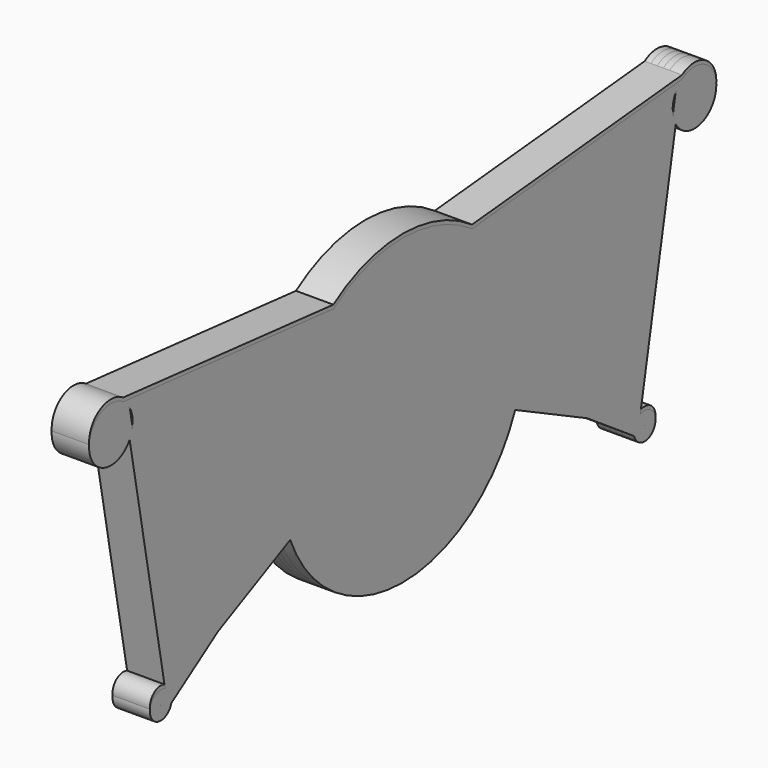
from build123d import *

# Parameters (mm, degrees)
F0_R     = 0.135
F0_R_2   = 0.27
F1_DEPTH = 25.4
F2_DEPTH = 6.35
F5_DEPTH = 12.7


# Not quite as in the source:
# - a feature of the source that left no trace in its solid (it failed there, or was rolled back) is left out


with BuildPart() as f1:
    # F0 (on Right) → F1 (new body)
    with BuildSketch(Plane.YZ):
        with BuildLine():
            ThreePointArc((148.1493894295, -44.1035673814), (152.9600066404, -22.2845823986), (154.5747917486, 0))
            ThreePointArc((154.5747917486, 0), (148.5279407682, 42.8114126754), (130.8604844604, 82.273324054))
            ThreePointArc((130.8604844604, 82.273324054), (111.8407913587, 106.700532484), (88.3348162489, 126.8476506775))
            ThreePointArc((88.3348162489, 126.8476506775), (0, 154.5747917486), (-88.3348162489, 126.8476506775))
            ThreePointArc((-88.3348162489, 126.8476506775), (-111.8407913587, 106.700532484), (-130.8604844604, 82.273324054))
            ThreePointArc((-130.8604844604, 82.273324054), (-153.1483173405, 20.9513517433), (-148.1493894296, -44.1035673814))
            ThreePointArc((-148.1493894296, -44.1035673814), (-145.885013799, -51.0972503466), (-143.2906938672, -57.9753680037))
            ThreePointArc((-143.2906938672, -57.9753680037), (0, -154.5747917486), (143.2906938672, -57.9753680037))
            ThreePointArc((143.2906938672, -57.9753680037), (145.885013799, -51.0972503466), (148.1493894295, -44.1035673814))
        make_face()
        with BuildLine():
            ThreePointArc((130.8604844604, 82.273324054), (148.5279407682, 42.8114126754), (154.5747917486, 0))
            ThreePointArc((154.5747917486, 0), (152.9600066404, -22.2845823986), (148.1493894295, -44.1035673814))
            Line((148.1493894296, -44.1035673814), (235.1719274058, -102.7744833812))
            Line((235.1719274058, -102.7744833812), (296.116428963, -132.4895802702))
            ThreePointArc((296.116428963, -132.4895802702), (296.5182456961, -131.8315982378), (296.9560527921, -131.1969944335))
            Line((296.9560527921, -131.1969944335), (344.4860615971, 123.2635601256))
            ThreePointArc((344.4860615971, 123.2635601256), (344.0765910751, 125.5101069455), (343.8526480641, 127.7826579901))
            Line((343.8526480641, 127.7826579901), (130.8604844604, 82.273324054))
        make_face()
        with BuildLine():
            ThreePointArc((88.3348162489, 126.8476506775), (111.8407913587, 106.700532484), (130.8604844604, 82.273324054))
            Line((130.8604844604, 82.273324054), (343.8526480641, 127.7826579901))
            ThreePointArc((343.8526480641, 127.7826579901), (344.791373956, 136.7102752623), (348.5227758692, 144.8748448298))
            ThreePointArc((348.5227758692, 144.8748448298), (351.8507398842, 148.9464286566), (355.885083858, 152.3194403742))
            Line((355.885083858, 152.3194403742), (88.3348162489, 126.8476506775))
        make_face()
        with BuildLine():
            Line((235.1719274058, -102.7744833812), (148.1493894296, -44.1035673814))
            ThreePointArc((148.1493894295, -44.1035673814), (145.885013799, -51.0972503466), (143.2906938672, -57.9753680037))
            Line((143.2906938672, -57.9753680037), (235.1719274058, -102.7744833812))
        make_face()
        with BuildLine():
            Line((296.116428963, -132.4895802702), (235.1719274058, -102.7744833812))
            Line((235.1719274058, -102.7744833812), (294.7499277685, -142.94219092))
            ThreePointArc((294.7499277685, -142.94219092), (294.3998362612, -137.5807936771), (296.116428963, -132.4895802702))
        make_face()
        with BuildLine():
            ThreePointArc((-130.8604844604, 82.273324054), (-111.8407913587, 106.700532484), (-88.3348162489, 126.8476506775))
            Line((-88.3348162489, 126.8476506775), (-355.885083858, 152.3194403742))
            ThreePointArc((-355.885083858, 152.3194403742), (-351.8507398842, 148.9464286566), (-348.5227758692, 144.8748448298))
            ThreePointArc((-348.5227758692, 144.8748448298), (-345.012126575, 137.4750271925), (-343.807133589, 129.3737957161))
            ThreePointArc((-343.807133589, 129.3737957161), (-343.8185145344, 128.5779014344), (-343.8526480641, 127.7826579901))
            Line((-343.8526480641, 127.7826579901), (-130.8604844604, 82.273324054))
        make_face()
        with BuildLine():
            ThreePointArc((399.477133589, 129.3737957161), (384.6072742696, 154.0049213934), (355.885083858, 152.3194403742))
            ThreePointArc((355.885083858, 152.3194403742), (351.8507398842, 148.9464286566), (348.5227758692, 144.8748448298))
            Line((348.5227758692, 144.8748448298), (344.4860615971, 123.2635601256))
            ThreePointArc((344.4860615971, 123.2635601256), (345.8076274671, 119.0120623456), (347.7901304496, 115.0256539813))
            ThreePointArc((347.7901304496, 115.0256539813), (379.0874917944, 102.5530226811), (399.477133589, 129.3737957161))
        make_face()
        with Locations((371.642133589, 129.3737957161)):
            Circle(F0_R, mode=Mode.SUBTRACT)
        with BuildLine():
            ThreePointArc((347.7901304496, 115.0256539813), (345.8076274671, 119.0120623456), (344.4860615971, 123.2635601256))
            Line((344.4860615971, 123.2635601256), (296.9560527921, -131.1969944335))
            ThreePointArc((296.9560527921, -131.1969944335), (299.4978488517, -128.5476375988), (302.6464556404, -126.6592271201))
            Line((302.6464556404, -126.6592271201), (347.7901304496, 115.0256539813))
        make_face()
        with BuildLine():
            Line((-235.1719274058, -102.7744833812), (-143.2906938672, -57.9753680037))
            ThreePointArc((-143.2906938672, -57.9753680037), (-145.885013799, -51.0972503466), (-148.1493894296, -44.1035673814))
            Line((-148.1493894295, -44.1035673814), (-235.1719274058, -102.7744833812))
        make_face()
        with BuildLine():
            ThreePointArc((296.9560527921, -131.1969944335), (296.5182456961, -131.8315982378), (296.116428963, -132.4895802702))
            ThreePointArc((296.116428963, -132.4895802702), (294.3998362612, -137.5807936771), (294.7499277685, -142.94219092))
            ThreePointArc((294.7499277685, -142.94219092), (309.9312086468, -153.1089342258), (321.9829761036, -139.3761683092))
            ThreePointArc((321.9829761036, -139.3761683092), (315.7433043352, -127.8044180436), (302.6464556404, -126.6592271201))
            ThreePointArc((302.6464556404, -126.6592271201), (299.4978488517, -128.5476375988), (296.9560527921, -131.1969944335))
        make_face()
        with Locations((308.1329761036, -139.3761683092)):
            Circle(F0_R_2, mode=Mode.SUBTRACT)
        with BuildLine():
            ThreePointArc((-148.1493894296, -44.1035673814), (-153.1483173405, 20.9513517433), (-130.8604844604, 82.273324054))
            Line((-130.8604844604, 82.273324054), (-343.8526480641, 127.7826579901))
            ThreePointArc((-343.8526480641, 127.7826579901), (-344.0765910751, 125.5101069455), (-344.4860615971, 123.2635601256))
            Line((-344.4860615971, 123.2635601256), (-296.9560527921, -131.1969944335))
            ThreePointArc((-296.9560527921, -131.1969944335), (-296.5182456961, -131.8315982378), (-296.116428963, -132.4895802702))
            Line((-296.116428963, -132.4895802702), (-235.1719274058, -102.7744833812))
            Line((-235.1719274058, -102.7744833812), (-148.1493894295, -44.1035673814))
        make_face()
        with BuildLine():
            ThreePointArc((-348.5227758692, 144.8748448298), (-351.8507398842, 148.9464286566), (-355.885083858, 152.3194403742))
            ThreePointArc((-355.885083858, 152.3194403742), (-398.8437124622, 123.4694471661), (-347.7901304496, 115.0256539813))
            ThreePointArc((-347.7901304496, 115.0256539813), (-345.8076274671, 119.0120623456), (-344.4860615971, 123.2635601256))
            Line((-344.4860615971, 123.2635601256), (-348.5227758692, 144.8748448298))
        make_face()
        with Locations((-371.642133589, 129.3737957161)):
            Circle(F0_R, mode=Mode.SUBTRACT)
        with BuildLine():
            Line((-294.7499277685, -142.94219092), (-235.1719274058, -102.7744833812))
            Line((-235.1719274058, -102.7744833812), (-296.116428963, -132.4895802702))
            ThreePointArc((-296.116428963, -132.4895802702), (-294.7491859473, -135.8129308695), (-294.2829761036, -139.3761683092))
            ThreePointArc((-294.2829761036, -139.3761683092), (-294.400210187, -141.1744008524), (-294.7499277685, -142.94219092))
        make_face()
        with BuildLine():
            ThreePointArc((-344.4860615971, 123.2635601256), (-345.8076274671, 119.0120623456), (-347.7901304496, 115.0256539813))
            Line((-347.7901304496, 115.0256539813), (-302.6464556404, -126.6592271201))
            ThreePointArc((-302.6464556404, -126.6592271201), (-299.4978488517, -128.5476375988), (-296.9560527921, -131.1969944335))
            Line((-296.9560527921, -131.1969944335), (-344.4860615971, 123.2635601256))
        make_face()
        with BuildLine():
            ThreePointArc((-302.6464556404, -126.6592271201), (-320.5948733984, -145.4196454386), (-294.7499277685, -142.94219092))
            ThreePointArc((-294.7499277685, -142.94219092), (-294.400210187, -141.1744008524), (-294.2829761036, -139.3761683092))
            ThreePointArc((-294.2829761036, -139.3761683092), (-294.7491859473, -135.8129308695), (-296.116428963, -132.4895802702))
            ThreePointArc((-296.116428963, -132.4895802702), (-296.5182456961, -131.8315982378), (-296.9560527921, -131.1969944335))
            ThreePointArc((-296.9560527921, -131.1969944335), (-299.4978488517, -128.5476375988), (-302.6464556404, -126.6592271201))
        make_face()
        with Locations((-308.1329761036, -139.3761683092)):
            Circle(F0_R_2, mode=Mode.SUBTRACT)
    extrude(amount=F1_DEPTH)

    # F0 (on Right) → F2 (join, symmetric)
    with BuildSketch(Plane.YZ):
        with BuildLine():
            ThreePointArc((148.1493894295, -44.1035673814), (152.9600066404, -22.2845823986), (154.5747917486, 0))
            ThreePointArc((154.5747917486, 0), (148.5279407682, 42.8114126754), (130.8604844604, 82.273324054))
            ThreePointArc((130.8604844604, 82.273324054), (111.8407913587, 106.700532484), (88.3348162489, 126.8476506775))
            ThreePointArc((88.3348162489, 126.8476506775), (0, 154.5747917486), (-88.3348162489, 126.8476506775))
            ThreePointArc((-88.3348162489, 126.8476506775), (-111.8407913587, 106.700532484), (-130.8604844604, 82.273324054))
            ThreePointArc((-130.8604844604, 82.273324054), (-153.1483173405, 20.9513517433), (-148.1493894296, -44.1035673814))
            ThreePointArc((-148.1493894296, -44.1035673814), (-145.885013799, -51.0972503466), (-143.2906938672, -57.9753680037))
            ThreePointArc((-143.2906938672, -57.9753680037), (0, -154.5747917486), (143.2906938672, -57.9753680037))
            ThreePointArc((143.2906938672, -57.9753680037), (145.885013799, -51.0972503466), (148.1493894295, -44.1035673814))
        make_face()
        with BuildLine():
            ThreePointArc((130.8604844604, 82.273324054), (148.5279407682, 42.8114126754), (154.5747917486, 0))
            ThreePointArc((154.5747917486, 0), (152.9600066404, -22.2845823986), (148.1493894295, -44.1035673814))
            Line((148.1493894296, -44.1035673814), (235.1719274058, -102.7744833812))
            Line((235.1719274058, -102.7744833812), (296.116428963, -132.4895802702))
            ThreePointArc((296.116428963, -132.4895802702), (296.5182456961, -131.8315982378), (296.9560527921, -131.1969944335))
            Line((296.9560527921, -131.1969944335), (344.4860615971, 123.2635601256))
            ThreePointArc((344.4860615971, 123.2635601256), (344.0765910751, 125.5101069455), (343.8526480641, 127.7826579901))
            Line((343.8526480641, 127.7826579901), (130.8604844604, 82.273324054))
        make_face()
        with BuildLine():
            ThreePointArc((88.3348162489, 126.8476506775), (111.8407913587, 106.700532484), (130.8604844604, 82.273324054))
            Line((130.8604844604, 82.273324054), (343.8526480641, 127.7826579901))
            ThreePointArc((343.8526480641, 127.7826579901), (344.791373956, 136.7102752623), (348.5227758692, 144.8748448298))
            ThreePointArc((348.5227758692, 144.8748448298), (351.8507398842, 148.9464286566), (355.885083858, 152.3194403742))
            Line((355.885083858, 152.3194403742), (88.3348162489, 126.8476506775))
        make_face()
        with BuildLine():
            Line((235.1719274058, -102.7744833812), (148.1493894296, -44.1035673814))
            ThreePointArc((148.1493894295, -44.1035673814), (145.885013799, -51.0972503466), (143.2906938672, -57.9753680037))
            Line((143.2906938672, -57.9753680037), (235.1719274058, -102.7744833812))
        make_face()
        with BuildLine():
            Line((296.116428963, -132.4895802702), (235.1719274058, -102.7744833812))
            Line((235.1719274058, -102.7744833812), (294.7499277685, -142.94219092))
            ThreePointArc((294.7499277685, -142.94219092), (294.3998362612, -137.5807936771), (296.116428963, -132.4895802702))
        make_face()
        with BuildLine():
            ThreePointArc((-130.8604844604, 82.273324054), (-111.8407913587, 106.700532484), (-88.3348162489, 126.8476506775))
            Line((-88.3348162489, 126.8476506775), (-355.885083858, 152.3194403742))
            ThreePointArc((-355.885083858, 152.3194403742), (-351.8507398842, 148.9464286566), (-348.5227758692, 144.8748448298))
            ThreePointArc((-348.5227758692, 144.8748448298), (-345.012126575, 137.4750271925), (-343.807133589, 129.3737957161))
            ThreePointArc((-343.807133589, 129.3737957161), (-343.8185145344, 128.5779014344), (-343.8526480641, 127.7826579901))
            Line((-343.8526480641, 127.7826579901), (-130.8604844604, 82.273324054))
        make_face()
        with BuildLine():
            ThreePointArc((399.477133589, 129.3737957161), (384.6072742696, 154.0049213934), (355.885083858, 152.3194403742))
            ThreePointArc((355.885083858, 152.3194403742), (351.8507398842, 148.9464286566), (348.5227758692, 144.8748448298))
            Line((348.5227758692, 144.8748448298), (344.4860615971, 123.2635601256))
            ThreePointArc((344.4860615971, 123.2635601256), (345.8076274671, 119.0120623456), (347.7901304496, 115.0256539813))
            ThreePointArc((347.7901304496, 115.0256539813), (379.0874917944, 102.5530226811), (399.477133589, 129.3737957161))
        make_face()
        with Locations((371.642133589, 129.3737957161)):
            Circle(F0_R, mode=Mode.SUBTRACT)
        with BuildLine():
            ThreePointArc((347.7901304496, 115.0256539813), (345.8076274671, 119.0120623456), (344.4860615971, 123.2635601256))
            Line((344.4860615971, 123.2635601256), (296.9560527921, -131.1969944335))
            ThreePointArc((296.9560527921, -131.1969944335), (299.4978488517, -128.5476375988), (302.6464556404, -126.6592271201))
            Line((302.6464556404, -126.6592271201), (347.7901304496, 115.0256539813))
        make_face()
        with BuildLine():
            Line((-235.1719274058, -102.7744833812), (-143.2906938672, -57.9753680037))
            ThreePointArc((-143.2906938672, -57.9753680037), (-145.885013799, -51.0972503466), (-148.1493894296, -44.1035673814))
            Line((-148.1493894295, -44.1035673814), (-235.1719274058, -102.7744833812))
        make_face()
        with BuildLine():
            ThreePointArc((296.9560527921, -131.1969944335), (296.5182456961, -131.8315982378), (296.116428963, -132.4895802702))
            ThreePointArc((296.116428963, -132.4895802702), (294.3998362612, -137.5807936771), (294.7499277685, -142.94219092))
            ThreePointArc((294.7499277685, -142.94219092), (309.9312086468, -153.1089342258), (321.9829761036, -139.3761683092))
            ThreePointArc((321.9829761036, -139.3761683092), (315.7433043352, -127.8044180436), (302.6464556404, -126.6592271201))
            ThreePointArc((302.6464556404, -126.6592271201), (299.4978488517, -128.5476375988), (296.9560527921, -131.1969944335))
        make_face()
        with Locations((308.1329761036, -139.3761683092)):
            Circle(F0_R_2, mode=Mode.SUBTRACT)
        with BuildLine():
            ThreePointArc((-148.1493894296, -44.1035673814), (-153.1483173405, 20.9513517433), (-130.8604844604, 82.273324054))
            Line((-130.8604844604, 82.273324054), (-343.8526480641, 127.7826579901))
            ThreePointArc((-343.8526480641, 127.7826579901), (-344.0765910751, 125.5101069455), (-344.4860615971, 123.2635601256))
            Line((-344.4860615971, 123.2635601256), (-296.9560527921, -131.1969944335))
            ThreePointArc((-296.9560527921, -131.1969944335), (-296.5182456961, -131.8315982378), (-296.116428963, -132.4895802702))
            Line((-296.116428963, -132.4895802702), (-235.1719274058, -102.7744833812))
            Line((-235.1719274058, -102.7744833812), (-148.1493894295, -44.1035673814))
        make_face()
        with BuildLine():
            ThreePointArc((-348.5227758692, 144.8748448298), (-351.8507398842, 148.9464286566), (-355.885083858, 152.3194403742))
            ThreePointArc((-355.885083858, 152.3194403742), (-398.8437124622, 123.4694471661), (-347.7901304496, 115.0256539813))
            ThreePointArc((-347.7901304496, 115.0256539813), (-345.8076274671, 119.0120623456), (-344.4860615971, 123.2635601256))
            Line((-344.4860615971, 123.2635601256), (-348.5227758692, 144.8748448298))
        make_face()
        with Locations((-371.642133589, 129.3737957161)):
            Circle(F0_R, mode=Mode.SUBTRACT)
        with BuildLine():
            Line((-294.7499277685, -142.94219092), (-235.1719274058, -102.7744833812))
            Line((-235.1719274058, -102.7744833812), (-296.116428963, -132.4895802702))
            ThreePointArc((-296.116428963, -132.4895802702), (-294.7491859473, -135.8129308695), (-294.2829761036, -139.3761683092))
            ThreePointArc((-294.2829761036, -139.3761683092), (-294.400210187, -141.1744008524), (-294.7499277685, -142.94219092))
        make_face()
        with BuildLine():
            ThreePointArc((-344.4860615971, 123.2635601256), (-345.8076274671, 119.0120623456), (-347.7901304496, 115.0256539813))
            Line((-347.7901304496, 115.0256539813), (-302.6464556404, -126.6592271201))
            ThreePointArc((-302.6464556404, -126.6592271201), (-299.4978488517, -128.5476375988), (-296.9560527921, -131.1969944335))
            Line((-296.9560527921, -131.1969944335), (-344.4860615971, 123.2635601256))
        make_face()
        with BuildLine():
            ThreePointArc((-302.6464556404, -126.6592271201), (-320.5948733984, -145.4196454386), (-294.7499277685, -142.94219092))
            ThreePointArc((-294.7499277685, -142.94219092), (-294.400210187, -141.1744008524), (-294.2829761036, -139.3761683092))
            ThreePointArc((-294.2829761036, -139.3761683092), (-294.7491859473, -135.8129308695), (-296.116428963, -132.4895802702))
            ThreePointArc((-296.116428963, -132.4895802702), (-296.5182456961, -131.8315982378), (-296.9560527921, -131.1969944335))
            ThreePointArc((-296.9560527921, -131.1969944335), (-299.4978488517, -128.5476375988), (-302.6464556404, -126.6592271201))
        make_face()
        with Locations((-308.1329761036, -139.3761683092)):
            Circle(F0_R_2, mode=Mode.SUBTRACT)
    extrude(amount=F2_DEPTH, both=True)

    # F0 (on Right) → F5 (join, symmetric)
    with BuildSketch(Plane.YZ):
        with BuildLine():
            ThreePointArc((148.1493894295, -44.1035673814), (152.9600066404, -22.2845823986), (154.5747917486, 0))
            ThreePointArc((154.5747917486, 0), (148.5279407682, 42.8114126754), (130.8604844604, 82.273324054))
            ThreePointArc((130.8604844604, 82.273324054), (111.8407913587, 106.700532484), (88.3348162489, 126.8476506775))
            ThreePointArc((88.3348162489, 126.8476506775), (0, 154.5747917486), (-88.3348162489, 126.8476506775))
            ThreePointArc((-88.3348162489, 126.8476506775), (-111.8407913587, 106.700532484), (-130.8604844604, 82.273324054))
            ThreePointArc((-130.8604844604, 82.273324054), (-153.1483173405, 20.9513517433), (-148.1493894296, -44.1035673814))
            ThreePointArc((-148.1493894296, -44.1035673814), (-145.885013799, -51.0972503466), (-143.2906938672, -57.9753680037))
            ThreePointArc((-143.2906938672, -57.9753680037), (0, -154.5747917486), (143.2906938672, -57.9753680037))
            ThreePointArc((143.2906938672, -57.9753680037), (145.885013799, -51.0972503466), (148.1493894295, -44.1035673814))
        make_face()
        with BuildLine():
            ThreePointArc((130.8604844604, 82.273324054), (148.5279407682, 42.8114126754), (154.5747917486, 0))
            ThreePointArc((154.5747917486, 0), (152.9600066404, -22.2845823986), (148.1493894295, -44.1035673814))
            Line((148.1493894296, -44.1035673814), (235.1719274058, -102.7744833812))
            Line((235.1719274058, -102.7744833812), (296.116428963, -132.4895802702))
            ThreePointArc((296.116428963, -132.4895802702), (296.5182456961, -131.8315982378), (296.9560527921, -131.1969944335))
            Line((296.9560527921, -131.1969944335), (344.4860615971, 123.2635601256))
            ThreePointArc((344.4860615971, 123.2635601256), (344.0765910751, 125.5101069455), (343.8526480641, 127.7826579901))
            Line((343.8526480641, 127.7826579901), (130.8604844604, 82.273324054))
        make_face()
        with BuildLine():
            ThreePointArc((88.3348162489, 126.8476506775), (111.8407913587, 106.700532484), (130.8604844604, 82.273324054))
            Line((130.8604844604, 82.273324054), (343.8526480641, 127.7826579901))
            ThreePointArc((343.8526480641, 127.7826579901), (344.791373956, 136.7102752623), (348.5227758692, 144.8748448298))
            ThreePointArc((348.5227758692, 144.8748448298), (351.8507398842, 148.9464286566), (355.885083858, 152.3194403742))
            Line((355.885083858, 152.3194403742), (88.3348162489, 126.8476506775))
        make_face()
        with BuildLine():
            Line((235.1719274058, -102.7744833812), (148.1493894296, -44.1035673814))
            ThreePointArc((148.1493894295, -44.1035673814), (145.885013799, -51.0972503466), (143.2906938672, -57.9753680037))
            Line((143.2906938672, -57.9753680037), (235.1719274058, -102.7744833812))
        make_face()
        with BuildLine():
            Line((296.116428963, -132.4895802702), (235.1719274058, -102.7744833812))
            Line((235.1719274058, -102.7744833812), (294.7499277685, -142.94219092))
            ThreePointArc((294.7499277685, -142.94219092), (294.3998362612, -137.5807936771), (296.116428963, -132.4895802702))
        make_face()
        with BuildLine():
            ThreePointArc((-130.8604844604, 82.273324054), (-111.8407913587, 106.700532484), (-88.3348162489, 126.8476506775))
            Line((-88.3348162489, 126.8476506775), (-355.885083858, 152.3194403742))
            ThreePointArc((-355.885083858, 152.3194403742), (-351.8507398842, 148.9464286566), (-348.5227758692, 144.8748448298))
            ThreePointArc((-348.5227758692, 144.8748448298), (-345.012126575, 137.4750271925), (-343.807133589, 129.3737957161))
            ThreePointArc((-343.807133589, 129.3737957161), (-343.8185145344, 128.5779014344), (-343.8526480641, 127.7826579901))
            Line((-343.8526480641, 127.7826579901), (-130.8604844604, 82.273324054))
        make_face()
        with BuildLine():
            ThreePointArc((399.477133589, 129.3737957161), (384.6072742696, 154.0049213934), (355.885083858, 152.3194403742))
            ThreePointArc((355.885083858, 152.3194403742), (351.8507398842, 148.9464286566), (348.5227758692, 144.8748448298))
            Line((348.5227758692, 144.8748448298), (344.4860615971, 123.2635601256))
            ThreePointArc((344.4860615971, 123.2635601256), (345.8076274671, 119.0120623456), (347.7901304496, 115.0256539813))
            ThreePointArc((347.7901304496, 115.0256539813), (379.0874917944, 102.5530226811), (399.477133589, 129.3737957161))
        make_face()
        with Locations((371.642133589, 129.3737957161)):
            Circle(F0_R, mode=Mode.SUBTRACT)
        with BuildLine():
            ThreePointArc((347.7901304496, 115.0256539813), (345.8076274671, 119.0120623456), (344.4860615971, 123.2635601256))
            Line((344.4860615971, 123.2635601256), (296.9560527921, -131.1969944335))
            ThreePointArc((296.9560527921, -131.1969944335), (299.4978488517, -128.5476375988), (302.6464556404, -126.6592271201))
            Line((302.6464556404, -126.6592271201), (347.7901304496, 115.0256539813))
        make_face()
        with BuildLine():
            Line((-235.1719274058, -102.7744833812), (-143.2906938672, -57.9753680037))
            ThreePointArc((-143.2906938672, -57.9753680037), (-145.885013799, -51.0972503466), (-148.1493894296, -44.1035673814))
            Line((-148.1493894295, -44.1035673814), (-235.1719274058, -102.7744833812))
        make_face()
        with BuildLine():
            ThreePointArc((296.9560527921, -131.1969944335), (296.5182456961, -131.8315982378), (296.116428963, -132.4895802702))
            ThreePointArc((296.116428963, -132.4895802702), (294.3998362612, -137.5807936771), (294.7499277685, -142.94219092))
            ThreePointArc((294.7499277685, -142.94219092), (309.9312086468, -153.1089342258), (321.9829761036, -139.3761683092))
            ThreePointArc((321.9829761036, -139.3761683092), (315.7433043352, -127.8044180436), (302.6464556404, -126.6592271201))
            ThreePointArc((302.6464556404, -126.6592271201), (299.4978488517, -128.5476375988), (296.9560527921, -131.1969944335))
        make_face()
        with Locations((308.1329761036, -139.3761683092)):
            Circle(F0_R_2, mode=Mode.SUBTRACT)
        with BuildLine():
            ThreePointArc((-148.1493894296, -44.1035673814), (-153.1483173405, 20.9513517433), (-130.8604844604, 82.273324054))
            Line((-130.8604844604, 82.273324054), (-343.8526480641, 127.7826579901))
            ThreePointArc((-343.8526480641, 127.7826579901), (-344.0765910751, 125.5101069455), (-344.4860615971, 123.2635601256))
            Line((-344.4860615971, 123.2635601256), (-296.9560527921, -131.1969944335))
            ThreePointArc((-296.9560527921, -131.1969944335), (-296.5182456961, -131.8315982378), (-296.116428963, -132.4895802702))
            Line((-296.116428963, -132.4895802702), (-235.1719274058, -102.7744833812))
            Line((-235.1719274058, -102.7744833812), (-148.1493894295, -44.1035673814))
        make_face()
        with BuildLine():
            ThreePointArc((-348.5227758692, 144.8748448298), (-351.8507398842, 148.9464286566), (-355.885083858, 152.3194403742))
            ThreePointArc((-355.885083858, 152.3194403742), (-398.8437124622, 123.4694471661), (-347.7901304496, 115.0256539813))
            ThreePointArc((-347.7901304496, 115.0256539813), (-345.8076274671, 119.0120623456), (-344.4860615971, 123.2635601256))
            Line((-344.4860615971, 123.2635601256), (-348.5227758692, 144.8748448298))
        make_face()
        with Locations((-371.642133589, 129.3737957161)):
            Circle(F0_R, mode=Mode.SUBTRACT)
        with BuildLine():
            Line((-294.7499277685, -142.94219092), (-235.1719274058, -102.7744833812))
            Line((-235.1719274058, -102.7744833812), (-296.116428963, -132.4895802702))
            ThreePointArc((-296.116428963, -132.4895802702), (-294.7491859473, -135.8129308695), (-294.2829761036, -139.3761683092))
            ThreePointArc((-294.2829761036, -139.3761683092), (-294.400210187, -141.1744008524), (-294.7499277685, -142.94219092))
        make_face()
        with BuildLine():
            ThreePointArc((-344.4860615971, 123.2635601256), (-345.8076274671, 119.0120623456), (-347.7901304496, 115.0256539813))
            Line((-347.7901304496, 115.0256539813), (-302.6464556404, -126.6592271201))
            ThreePointArc((-302.6464556404, -126.6592271201), (-299.4978488517, -128.5476375988), (-296.9560527921, -131.1969944335))
            Line((-296.9560527921, -131.1969944335), (-344.4860615971, 123.2635601256))
        make_face()
        with BuildLine():
            ThreePointArc((-302.6464556404, -126.6592271201), (-320.5948733984, -145.4196454386), (-294.7499277685, -142.94219092))
            ThreePointArc((-294.7499277685, -142.94219092), (-294.400210187, -141.1744008524), (-294.2829761036, -139.3761683092))
            ThreePointArc((-294.2829761036, -139.3761683092), (-294.7491859473, -135.8129308695), (-296.116428963, -132.4895802702))
            ThreePointArc((-296.116428963, -132.4895802702), (-296.5182456961, -131.8315982378), (-296.9560527921, -131.1969944335))
            ThreePointArc((-296.9560527921, -131.1969944335), (-299.4978488517, -128.5476375988), (-302.6464556404, -126.6592271201))
        make_face()
        with Locations((-308.1329761036, -139.3761683092)):
            Circle(F0_R_2, mode=Mode.SUBTRACT)
    extrude(amount=F5_DEPTH, both=True)


with BuildPart() as f6_1:
    # F6: copy of F1
    add(f1.part.moved(Location((0, 0, -3.81))))


solid = Compound([f1.part, f6_1.part])
